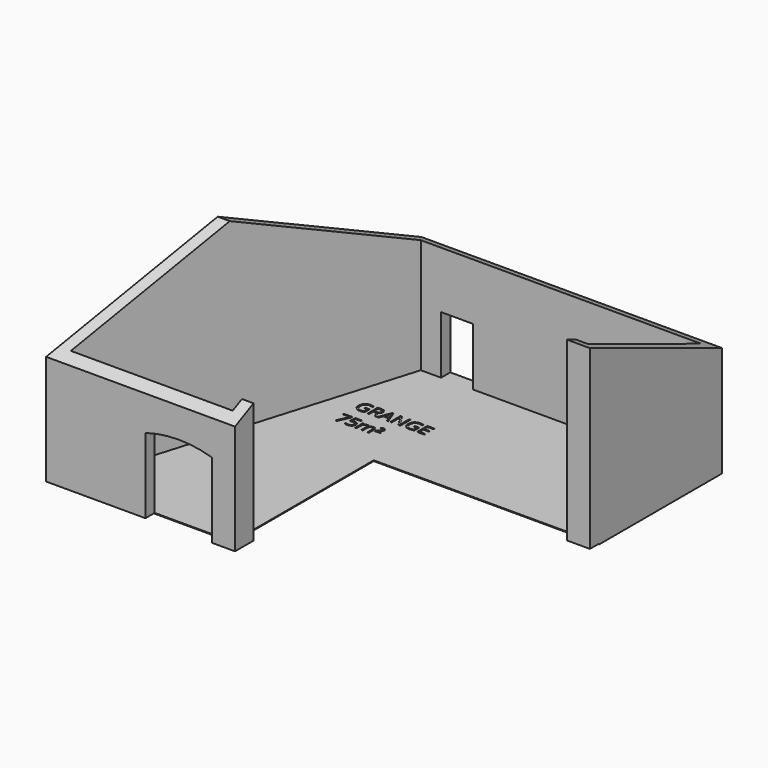
from build123d import *

# Parameters (mm, degrees)
F1_DEPTH      = 6400
F3_DEPTH      = 400.001
F3_DEPTH_BACK = 13537.4729630096
F4_W          = 1100
F4_H          = 2000
F5_DEPTH      = 400
F7_DEPTH      = 400
F9_DEPTH      = 1
F9_DEPTH_BACK = 25
F10_TEXT_SIZE = 627.6802884208
F11_DEPTH     = 25


# Not quite as in the source:
# - Text() gives the source's letters only with a copy of the font that has no kerning and outlines rounded to 1/6400 em; it was checked with that copy


with BuildPart() as f1:
    # F0 (on Top) → F1 (new body)
    with BuildSketch(Plane.XY):
        Polygon((-13000, -6100), (-9700, 4910), (0, 4910), (0, 0), (-400, 0), (-400, -400), (400, -400), (400, 5310), (-9997.6899466608, 5310), (-13537.4719630096, -6500), (-7000, -6500), (-7000, -5700), (-7400, -5700), (-7400, -6100), align=None)
    extrude(amount=F1_DEPTH)

    # F2 (on Right) → F3 (cut, two sides)
    with BuildSketch(Plane.YZ) as f3_sk:
        Polygon((-6500, 6400), (-6500, 3800), (-1100, 6400), align=None)
        Polygon((5310, 6400), (-1100, 6400), (5310, 3800), align=None)
    extrude(amount=F3_DEPTH, mode=Mode.SUBTRACT)
    extrude(f3_sk.sketch, amount=-F3_DEPTH_BACK, mode=Mode.SUBTRACT)

    # F4 (on face) → F5 (cut, through all)
    with BuildSketch(Plane(origin=(0, 5310, 0), x_dir=(-1, 0, 0), z_dir=(0, 1, 0))):
        with Locations((8447.6899466608, 1000)):
            Rectangle(F4_W, F4_H)
    extrude(amount=-F5_DEPTH, mode=Mode.SUBTRACT)

    # F6 (on face) → F7 (cut, through all)
    with BuildSketch(Plane.XZ.offset(6500)):
        with BuildLine():
            Line((-10100, 2600), (-10100, 0))
            Line((-10100, 0), (-7800, 0))
            Line((-7800, 0), (-7800, 2600))
            ThreePointArc((-7800, 2600), (-8950, 2768.8774491019), (-10100, 2600))
        make_face()
    extrude(amount=-F7_DEPTH, mode=Mode.SUBTRACT)

    # F8 (on face) → F9 (join, two sides)
    with BuildSketch(Plane(origin=(0, 0, 0), x_dir=(1, 0, 0), z_dir=(0, 0, -1))) as f9_sk:
        Polygon((-13417.5809548352, 6100), (-9997.6899466608, -5310), (400, -5310), (400, 0), (-7400, 0), (-7400, 6100), align=None)
    extrude(amount=-F9_DEPTH)
    extrude(f9_sk.sketch, amount=F9_DEPTH_BACK)

    # F10 (on face) → F11 (cut)
    with BuildSketch(Plane.XY.offset(1)):
        with Locations((-9757.9562664032, 2026.2234210968)):
            Text('GRANGE', F10_TEXT_SIZE, font='Open Sans', text_align=(TextAlign.LEFT, TextAlign.BOTTOM))
        with Locations((-9757.9562664032, 1172.5782288445)):
            Text('75m²', F10_TEXT_SIZE, font='Open Sans', text_align=(TextAlign.LEFT, TextAlign.BOTTOM))
    extrude(amount=-F11_DEPTH, mode=Mode.SUBTRACT)


solid = f1.part
